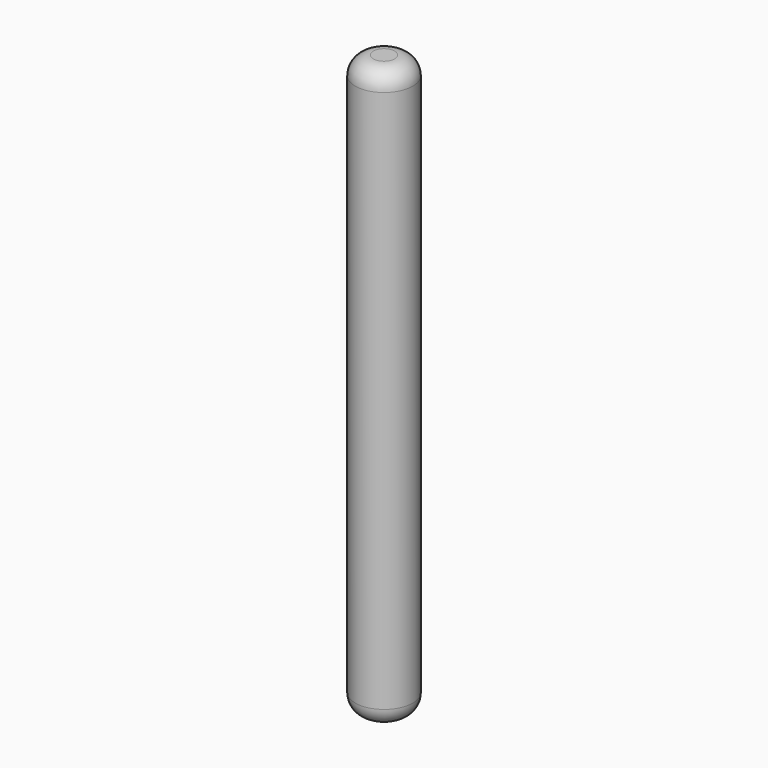
from build123d import *

# Parameters (mm, degrees)
F3_R     = 1.5875
F4_DEPTH = 32
F5_R     = 1


with BuildPart() as f4:
    # F3 (on Top) → F4 (new body)
    with BuildSketch(Plane.XY):
        Circle(F3_R)
    extrude(amount=F4_DEPTH)

    # F5
    f5_edges = [f4.edges().sort_by_distance(p)[0] for p in [
        (-1.5875, 0, 32),
        (-1.5875, 0, 0),
    ]]
    fillet(f5_edges, radius=F5_R)


solid = f4.part
